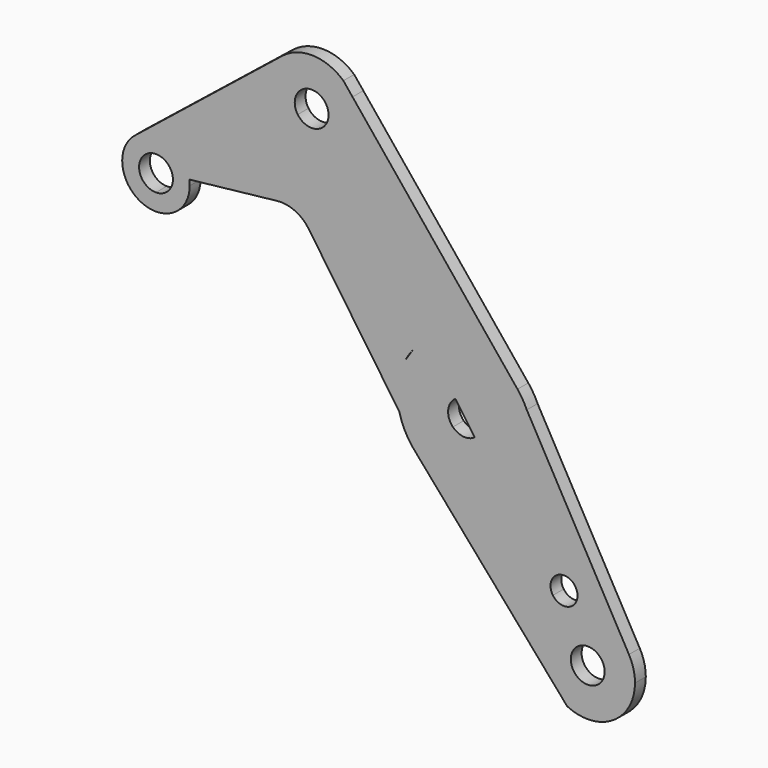
from build123d import *

# Parameters (mm, degrees)
F1_DEPTH = 3.175


# Not quite as in the source:
# - a feature names something its author has since deleted; it is built from what else it names


with BuildPart() as f1:
    # F0 (on Front) → F1 (new body)
    with BuildSketch(Plane.XZ):
        with BuildLine():
            ThreePointArc((41.2067680932, -37.761442646), (34.0261463641, -32.3730062039), (25.2065586875, -34.049743787))
            ThreePointArc((25.2065586875, -34.049743787), (20.9962687571, -39.6141258639), (20.9333080978, -46.5915842229))
            Line((20.9333080978, -46.5915842229), (26.6775649821, -53.2024105477))
            ThreePointArc((26.6775649821, -53.2024105477), (37.4197145601, -52.6119623059), (42.6274718911, -43.1980539644))
            ThreePointArc((42.6274718911, -43.1980539644), (42.2664308978, -40.3884658314), (41.2067680932, -37.761442646))
        make_face()
        with BuildLine():
            ThreePointArc((35.4900718911, -43.1980539644), (29.6668415528, -46.7174053624), (29.258362368, -39.9255727238))
            ThreePointArc((29.258362368, -39.9255727238), (33.3631022294, -39.6787025664), (35.4900718911, -43.1980539644))
        make_face(mode=Mode.SUBTRACT)
        with BuildLine():
            ThreePointArc((20.9333080978, -46.5915842229), (20.9962687571, -39.6141258639), (25.2065586875, -34.049743787))
            Line((25.2065586875, -34.049743787), (23.332877686, -31.3325763437))
            Line((23.332877686, -31.3325763437), (11.7179656145, -14.4889082319))
            Line((11.7179656145, -14.4889082319), (0.788153606, -23.4073638243))
            Line((0.788153606, -23.4073638243), (20.9333080978, -46.5915842229))
        make_face()
        with BuildLine():
            Line((23.332877686, -31.3325763437), (25.2065586875, -34.049743787))
            ThreePointArc((25.2065586875, -34.049743787), (34.0261463641, -32.3730062039), (41.2067680932, -37.761442646))
            Line((41.2067680932, -37.761442646), (17.1943117559, 5.0453389137))
            ThreePointArc((17.1943117559, 5.0453389137), (18.2085059877, 1.9049828695), (18.5515115318, -1.377207439))
            ThreePointArc((18.5515115318, -1.377207439), (17.0177668978, -8.1848516369), (12.7128948986, -13.6770706055))
            Line((12.7128948986, -13.6770706055), (11.7179656145, -14.4889082319))
            Line((11.7179656145, -14.4889082319), (23.332877686, -31.3325763437))
        make_face()
        with BuildLine():
            ThreePointArc((29.1216807586, -29.5301728102), (26.8905558151, -32.5616287109), (23.332877686, -31.3325763437))
            ThreePointArc((23.332877686, -31.3325763437), (25.0028057021, -26.4987169095), (29.1216807586, -29.5301728102))
        make_face(mode=Mode.SUBTRACT)
        with BuildLine():
            Line((0.788153606, -23.4073638243), (11.7179656145, -14.4889082319))
            Line((11.7179656145, -14.4889082319), (11.6885303941, -14.4462219782))
            ThreePointArc((11.6885303941, -14.4462219782), (1.1239010077, -17.1761006141), (-8.7072046251, -12.4418643003))
            Line((-8.7072046251, -12.4418643003), (-8.7249576565, -12.4591197552))
            Line((-8.7249576565, -12.4591197552), (0.788153606, -23.4073638243))
        make_face()
        with BuildLine():
            Line((11.6885303941, -14.4462219782), (11.7179656145, -14.4889082319))
            Line((11.7179656145, -14.4889082319), (12.7128948986, -13.6770706055))
            ThreePointArc((12.7128948986, -13.6770706055), (12.2084738339, -14.0719827293), (11.6885303941, -14.4462219782))
        make_face()
        with BuildLine():
            ThreePointArc((18.5515115318, -1.377207439), (18.2085059877, 1.9049828695), (17.1943117559, 5.0453389137))
            ThreePointArc((17.1943117559, 5.0453389137), (16.2212708068, 6.9025945623), (15.0119525687, 8.6154158115))
            ThreePointArc((15.0119525687, 8.6154158115), (4.9408722756, 14.3354720086), (-6.3355073305, 11.6918071002))
            Line((-6.3355073305, 11.6918071002), (0.4199020087, 1.8952738016))
            ThreePointArc((0.4199020087, 1.8952738016), (4.5246418701, 2.142143959), (6.6516115318, -1.377207439))
            ThreePointArc((6.6516115318, -1.377207439), (6.1958629298, -3.2253377773), (4.9331210549, -4.6496886796))
            Line((4.9331210549, -4.6496886796), (11.6885303941, -14.4462219782))
            ThreePointArc((11.6885303941, -14.4462219782), (12.2084738339, -14.0719827293), (12.7128948986, -13.6770706055))
            ThreePointArc((12.7128948986, -13.6770706055), (17.0177668978, -8.1848516369), (18.5515115318, -1.377207439))
        make_face()
        with BuildLine():
            ThreePointArc((-8.7072046251, -12.4418643003), (1.1239010077, -17.1761006141), (11.6885303941, -14.4462219782))
            Line((11.6885303941, -14.4462219782), (4.9331210549, -4.6496886796))
            ThreePointArc((4.9331210549, -4.6496886796), (2.2877378565, -5.33325029), (-0.1739709939, -4.147797517))
            Line((-0.1739709939, -4.147797517), (-8.7072046251, -12.4418643003))
        make_face()
        with BuildLine():
            ThreePointArc((-6.3355073305, 11.6918071002), (4.9408722756, 14.3354720086), (15.0119525687, 8.6154158115))
            Line((15.0119525687, 8.6154158115), (-23.7631885124, 56.4815721265))
            ThreePointArc((-23.7631885124, 56.4815721265), (-22.6416820928, 53.7897488967), (-22.2590639174, 50.8988507178))
            ThreePointArc((-22.2590639174, 50.8988507178), (-23.5331215108, 45.7323521683), (-27.0631507138, 41.7505405404))
            Line((-27.0631507138, 41.7505405404), (-6.3355073305, 11.6918071002))
        make_face()
        with BuildLine():
            Line((2.6765115318, -1.377207439), (4.9331210549, -4.6496886796))
            ThreePointArc((4.9331210549, -4.6496886796), (6.1958629298, -3.2253377773), (6.6516115318, -1.377207439))
            ThreePointArc((6.6516115318, -1.377207439), (4.5246418701, 2.142143959), (0.4199020087, 1.8952738016))
            Line((0.4199020087, 1.8952738016), (2.6765115318, -1.377207439))
        make_face()
        with BuildLine():
            ThreePointArc((-12.7591425966, -5.0861434898), (-11.2283909413, -9.0367969981), (-8.7072046251, -12.4418643003))
            Line((-8.7072046251, -12.4418643003), (-0.1739709939, -4.147797517))
            ThreePointArc((-0.1739709939, -4.147797517), (-1.2795313193, -0.9884337637), (0.4199020087, 1.8952738016))
            Line((0.4199020087, 1.8952738016), (-6.3355073305, 11.6918071002))
            ThreePointArc((-6.3355073305, 11.6918071002), (-8.12621733, 10.2553621026), (-9.6910264168, 8.5756630059))
            Line((-9.6910264168, 8.5756630059), (-11.3706653491, 6.0182267388))
            ThreePointArc((-11.3706653491, 6.0182267388), (-13.0758245053, 0.5924459256), (-12.7591425966, -5.0861434898))
        make_face()
        with BuildLine():
            ThreePointArc((-9.6910264168, 8.5756630059), (-8.12621733, 10.2553621026), (-6.3355073305, 11.6918071002))
            Line((-6.3355073305, 11.6918071002), (-27.0631507138, 41.7505405404))
            ThreePointArc((-27.0631507138, 41.7505405404), (-35.3796743255, 39.9692968001), (-42.5198740948, 44.5904375142))
            Line((-42.5198740948, 44.5904375142), (-63.4302973575, 30.1712073345))
            ThreePointArc((-63.4302973575, 30.1712073345), (-62.5957178566, 28.6148532084), (-62.125916075, 26.9124879729))
            Line((-62.125916075, 26.9124879729), (-41.4863105467, 29.2003405071))
            ThreePointArc((-41.4863105467, 29.2003405071), (-37.3081114888, 28.5304448001), (-34.0654515171, 25.8117568934))
            Line((-34.0654515171, 25.8117568934), (-15.783328424, -0.7005414231))
            Line((-15.783328424, -0.7005414231), (-11.3706653491, 6.0182267388))
            ThreePointArc((-11.3706653491, 6.0182267388), (-10.5926033575, 7.337505124), (-9.6910264168, 8.5756630059))
        make_face()
        with BuildLine():
            ThreePointArc((-22.2590639174, 50.8988507178), (-22.6416820928, 53.7897488967), (-23.7631885124, 56.4815721265))
            Line((-23.7631885124, 56.4815721265), (-25.9160326978, 59.1391608141))
            ThreePointArc((-25.9160326978, 59.1391608141), (-33.0370839347, 62.0063157477), (-40.3177534576, 59.572840983))
            ThreePointArc((-40.3177534576, 59.572840983), (-44.3659412857, 52.514809422), (-42.5198740948, 44.5904375142))
            Line((-42.5198740948, 44.5904375142), (-36.644045158, 48.6422411947))
            ThreePointArc((-36.644045158, 48.6422411947), (-34.5532956616, 54.6942334514), (-29.3964639174, 50.8988507178))
            ThreePointArc((-29.3964639174, 50.8988507178), (-29.8522125194, 49.0507203795), (-31.1149543943, 47.6263694772))
            Line((-31.1149543943, 47.6263694772), (-27.0631507138, 41.7505405404))
            ThreePointArc((-27.0631507138, 41.7505405404), (-23.5331215108, 45.7323521683), (-22.2590639174, 50.8988507178))
        make_face()
        with BuildLine():
            Line((-15.783328424, -0.7005414231), (-12.7591425966, -5.0861434898))
            ThreePointArc((-12.7591425966, -5.0861434898), (-13.0758245053, 0.5924459256), (-11.3706653491, 6.0182267388))
            Line((-11.3706653491, 6.0182267388), (-15.783328424, -0.7005414231))
        make_face()
        with BuildLine():
            ThreePointArc((-42.5198740948, 44.5904375142), (-35.3796743255, 39.9692968001), (-27.0631507138, 41.7505405404))
            Line((-27.0631507138, 41.7505405404), (-31.1149543943, 47.6263694772))
            ThreePointArc((-31.1149543943, 47.6263694772), (-34.0898936977, 46.989193145), (-36.644045158, 48.6422411947))
            Line((-36.644045158, 48.6422411947), (-42.5198740948, 44.5904375142))
        make_face()
        with BuildLine():
            Line((-63.4302973575, 30.1712073345), (-42.5198740948, 44.5904375142))
            ThreePointArc((-42.5198740948, 44.5904375142), (-44.3659412857, 52.514809422), (-40.3177534576, 59.572840983))
            Line((-40.3177534576, 59.572840983), (-74.7776425006, 31.9771308762))
            ThreePointArc((-74.7776425006, 31.9771308762), (-68.717256497, 33.5040453897), (-63.4302973575, 30.1712073345))
        make_face()
        with BuildLine():
            ThreePointArc((-62.125916075, 26.9124879729), (-62.5957178566, 28.6148532084), (-63.4302973575, 30.1712073345))
            Line((-63.4302973575, 30.1712073345), (-66.6923233865, 27.9218074265))
            ThreePointArc((-66.6923233865, 27.9218074265), (-66.1694218935, 26.8469296476), (-65.9897046271, 25.6651979034))
            ThreePointArc((-65.9897046271, 25.6651979034), (-67.1539844612, 22.8543777375), (-69.9648046271, 21.6900979034))
            Line((-69.9648046271, 21.6900979034), (-69.9648046271, 17.7276979034))
            ThreePointArc((-69.9648046271, 17.7276979034), (-64.3521445515, 20.0525378277), (-62.0273046271, 25.6651979034))
            ThreePointArc((-62.0273046271, 25.6651979034), (-62.0519958928, 26.2907889709), (-62.125916075, 26.9124879729))
        make_face()
        with BuildLine():
            Line((-66.6923233865, 27.9218074265), (-63.4302973575, 30.1712073345))
            ThreePointArc((-63.4302973575, 30.1712073345), (-68.717256497, 33.5040453897), (-74.7776425006, 31.9771308762))
            Line((-74.7776425006, 31.9771308762), (-75.0722889717, 31.7411760073))
            ThreePointArc((-75.0722889717, 31.7411760073), (-77.4224175981, 22.9471259719), (-69.9648046271, 17.7276979034))
            Line((-69.9648046271, 17.7276979034), (-69.9648046271, 21.6900979034))
            ThreePointArc((-69.9648046271, 21.6900979034), (-73.4841560252, 27.5133282417), (-66.6923233865, 27.9218074265))
        make_face()
    extrude(amount=F1_DEPTH)


solid = f1.part
